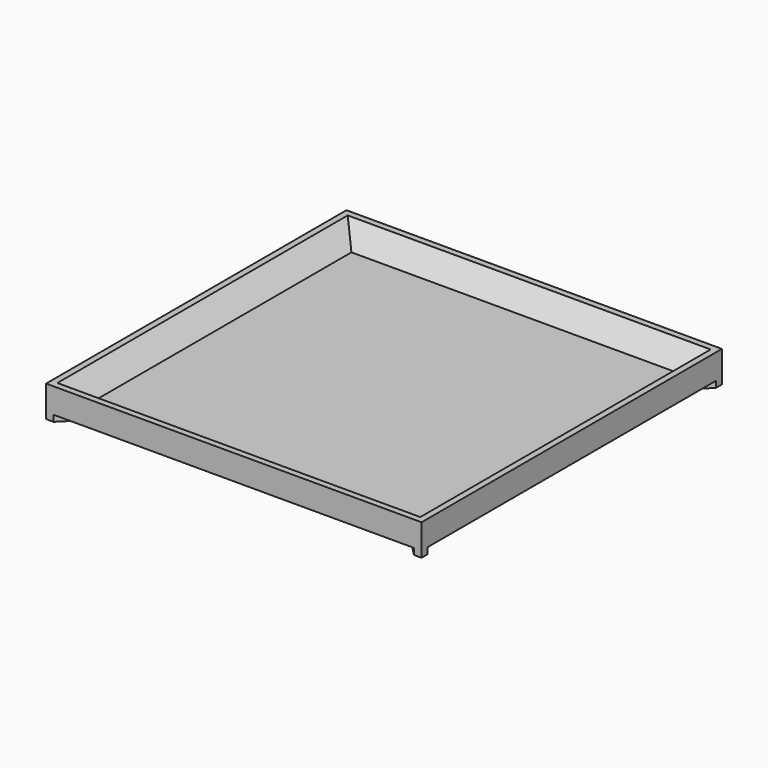
from build123d import *

# Parameters (mm, degrees)
F0_W     = 150
F0_H     = 150
F1_DEPTH = 10
F2_T     = -2.5
F3_SIZE  = 7.49999
F5_DEPTH = 2.5


# Not quite as in the source:
# - a fillet or chamfer is up to 0.001 mm smaller than in the source, because OpenCascade refuses the exact size


with BuildPart() as f1:
    # F0 (on Top) → F1 (new body)
    with BuildSketch(Plane.XY):
        Rectangle(F0_W, F0_H)
    extrude(amount=F1_DEPTH)

    # F2
    f2_openings = [f1.faces().sort_by_distance(p)[0] for p in [
        (0, 0, 10),
    ]]
    offset(amount=F2_T, openings=f2_openings)

    # F3 (size 7.5 in the source; OpenCascade refuses exactly that, so slightly less here)
    f3_edges = [f1.edges().sort_by_distance(p)[0] for p in [
        (-72.5, 0, 2.5),
        (0, 72.5, 2.5),
        (72.5, 0, 2.5),
        (0, -72.5, 2.5),
    ]]
    chamfer(f3_edges, length=F3_SIZE)

    # F4 (on face) → F5 (join)
    with BuildSketch(Plane(origin=(0, 0, 0), x_dir=(1, 0, 0), z_dir=(0, 0, -1))):
        Polygon((0, 3), (-72, 75), (-75, 75), (-75, 72), (-3, 0), (-75, -72), (-75, -75), (-72, -75), (0, -3), (72, -75), (75, -75), (75, -72), (3, 0), (75, 72), (75, 75), (72, 75), align=None)
    extrude(amount=F5_DEPTH)


solid = f1.part
